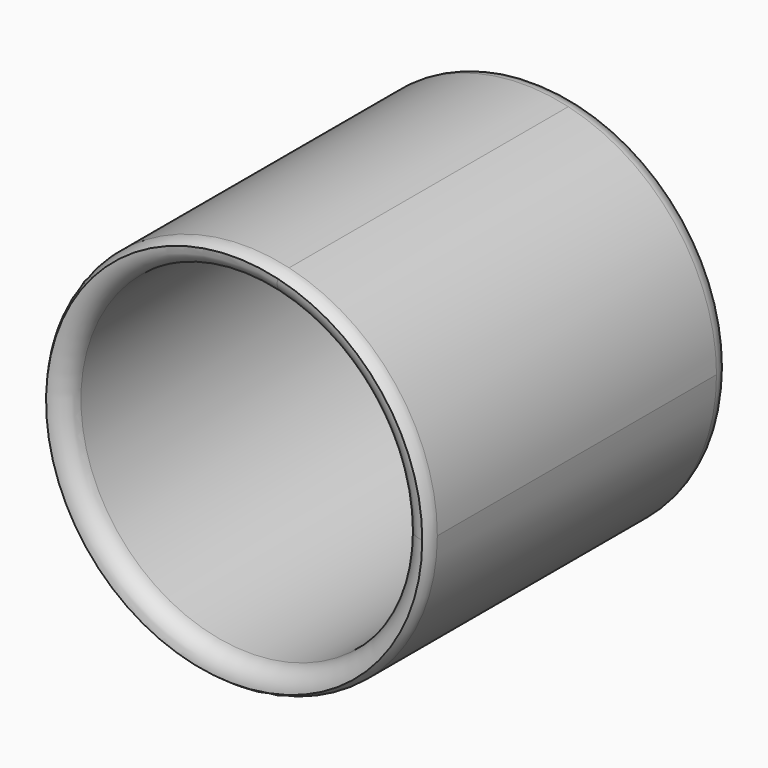
from build123d import *

# Parameters (mm, degrees)
F1_DEPTH = 98.21704
F2_R     = 5.08
F4_R     = 5.08


# Not quite as in the source:
# - a fillet or chamfer that OpenCascade refuses, or shapes differently, is made with other operations: its cross-section is extruded or revolved along the edge and cut away or added


with BuildPart() as f1:
    # F0 (on Front) → F1 (new body)
    with BuildSketch(Plane.XZ):
        with BuildLine():
            ThreePointArc((11.7319880136, 49.2156378568), (-39.7076464503, -31.3547662371), (50.5946494444, 0))
            ThreePointArc((50.5946494444, 0), (39.7076464503, 31.3547662371), (11.7319880136, 49.2156378568))
        make_face()
        with BuildLine():
            ThreePointArc((44.2446494444, 0), (-34.7240452646, -27.4195128498), (10.2595373749, 43.0387139366))
            ThreePointArc((10.2595373749, 43.0387139366), (34.7240452646, 27.4195128498), (44.2446494444, 0))
        make_face(mode=Mode.SUBTRACT)
    extrude(amount=F1_DEPTH)

    # F2
    f2_edges = [f1.edges().sort_by_distance(p)[0] for p in [
        (-10.259537, -98.21704, -43.038714),
    ]]
    fillet(f2_edges, radius=F2_R)

    # F3: fillet of radius 5.08 on 1 edges, made by hand

    # F3_s1 → F3_t2 (revolve, cut)
    with BuildSketch(Plane.XY):
        with BuildLine():
            ThreePointArc((49.3246494444, -98.21704), (50.2665543256, -96.6529870592), (50.5946494444, -94.8569358349))
            Line((50.5946494444, -94.8569358349), (50.5946494444, -98.21704))
            Line((50.5946494444, -98.21704), (49.3246494444, -98.21704))
        make_face()
    revolve(axis=Axis((0, -98.21704, 0), (0, 1, 0)), mode=Mode.SUBTRACT)

    # F4
    f4_edges = [f1.edges().sort_by_distance(p)[0] for p in [
        (-10.259537, 0, -43.038714),
    ]]
    fillet(f4_edges, radius=F4_R)

    # F5: fillet of radius 5.08 on 1 edges, made by hand

    # F5_s1 → F5_t2 (revolve, cut)
    with BuildSketch(Plane.XY):
        with BuildLine():
            ThreePointArc((49.3246494444, 0), (50.2665543256, -1.5640529408), (50.5946494444, -3.3601041651))
            Line((50.5946494444, -3.3601041651), (50.5946494444, 0))
            Line((50.5946494444, 0), (49.3246494444, 0))
        make_face()
    revolve(axis=Axis((0, 0, 0), (0, -1, 0)), mode=Mode.SUBTRACT)


solid = f1.part
